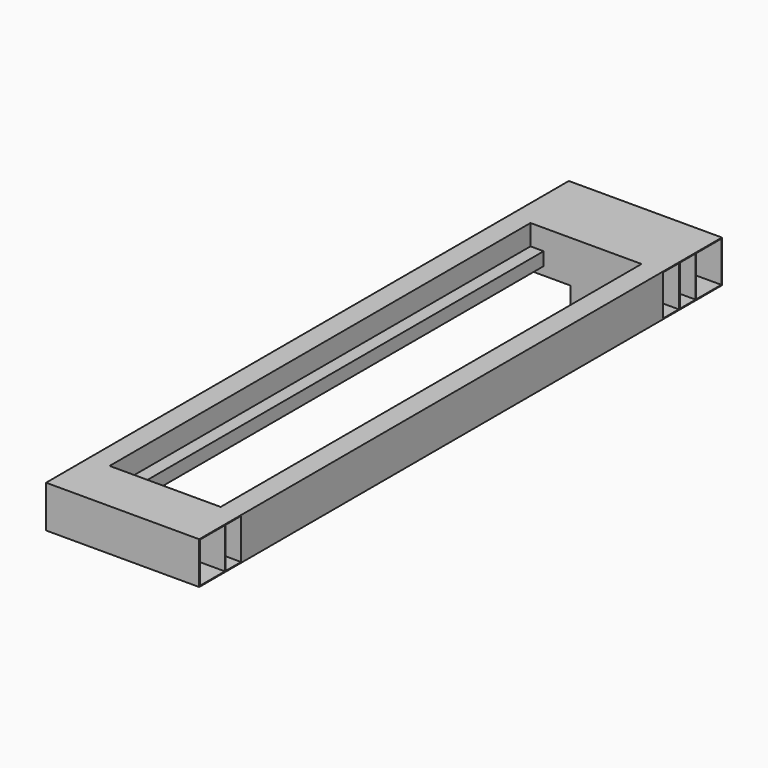
from build123d import *

# Parameters (mm, degrees)
F0_W      = 74
F0_H      = 154
F0_W_2    = 46
F0_H_2    = 46
F1_DEPTH  = 2000
F6_W      = 74
F6_H      = 154
F7_DEPTH  = 582
F8_W      = 74
F8_H      = 154
F9_DEPTH  = 582
F10_W     = 58.25
F10_H     = 30.13
F11_DEPTH = 2160.001
F12_W     = 116.5
F12_H     = 3
F13_DEPTH = 74
F14_W     = 116.5
F14_H     = 3
F15_DEPTH = 76
F16_W     = 116.5
F16_H     = 3
F17_DEPTH = 71
F18_W     = 116.5
F18_H     = 3
F19_DEPTH = 95
F20_W     = 116.5
F20_H     = 3
F20_H_2   = 22.57
F21_DEPTH = 77
F22_DEPTH = 77
F23_DEPTH = 77
F24_W     = 74
F24_H     = 154
F25_DEPTH = 582
F27_DEPTH = 3
F29_DEPTH = 582
F31_DEPTH = 25
F32_DEPTH = 582
F34_DEPTH = 25


# Not quite as in the source:
# - a feature names something its author has since deleted; it is built from what else it names


with BuildPart() as f1:
    # F0 (on Front) → F1 (new body)
    with BuildSketch(Plane.XZ):
        Polygon((-80, 0), (0, 0), (0, 16.85), (0, 31.78), (0, 81.78), (0, 160), (-77, 160), (-80, 160), align=None)
        with Locations((-40, 80)):
            Rectangle(F0_W, F0_H, mode=Mode.SUBTRACT)
        Polygon((0, 81.78), (0, 31.78), (50, 31.78), (50, 81.78), (2, 81.78), align=None)
        with Locations((25, 56.78)):
            Rectangle(F0_W_2, F0_H_2, mode=Mode.SUBTRACT)
    extrude(amount=F1_DEPTH)


with BuildPart() as f2_1:
    # F2: instance of F1
    add(f1.part.mirror(Plane(origin=(50, -1000, 56.78), x_dir=(0, 1, 0), z_dir=(1, 0, 0))))


with BuildPart() as f2_1_1:
    # F3: moved
    add(f2_1.part.moved(Location((63, 0, 0))))


with BuildPart() as f2_1_2:
    # F5: moved
    add(f2_1_1.part.moved(Location((259.1, 0, 0))))


with BuildPart() as f1_1:
    add(f1.part)

    add(f2_1_2.part)  # F7 merges F2_1
    # F6 (on face) → F7 (join)
    with BuildSketch(Plane.YZ.offset(502.1)):
        Polygon((-2000, 0), (-2000, 160), (-2077, 160), (-2080, 160), (-2080, 0), align=None)
        with Locations((-2040, 80)):
            Rectangle(F6_W, F6_H, mode=Mode.SUBTRACT)
    extrude(amount=-F7_DEPTH)

    # F8 (on face) → F9 (join)
    with BuildSketch(Plane.YZ.offset(502.1)):
        Polygon((80, 160), (0, 160), (0, 0), (3, 0), (80, 0), align=None)
        with Locations((40, 80)):
            Rectangle(F8_W, F8_H, mode=Mode.SUBTRACT)
    extrude(amount=-F9_DEPTH)

    # F10 (on face) → F11 (cut, through all)
    with BuildSketch(Plane.XZ.offset(2080)):
        with Locations((182.125, 15.065)):
            Rectangle(F10_W, F10_H)
        with Locations((240.375, 15.065)):
            Rectangle(F10_W, F10_H)
    extrude(amount=-F11_DEPTH, mode=Mode.SUBTRACT)

    # F12 (on face) + F10 (on face) → F13 (join)
    with BuildSketch(Plane(origin=(0, -2077, 0), x_dir=(-1, 0, 0), z_dir=(0, 1, 0))):
        with Locations((-211.25, 31.63)):
            Rectangle(F12_W, F12_H)
    with BuildSketch(Plane.XZ.offset(2080)):
        with Locations((182.125, 15.065)):
            Rectangle(F10_W, F10_H)
    extrude(amount=F13_DEPTH, dir=(0, 1, 0))

    # F14 (on face) → F15 (join)
    with BuildSketch(Plane.XZ.offset(-77)):
        with Locations((211.25, 31.63)):
            Rectangle(F14_W, F14_H)
    extrude(amount=F15_DEPTH)

    # F16 (on face) → F17 (join)
    with BuildSketch(Plane(origin=(0, 0, 30.13), x_dir=(1, 0, 0), z_dir=(0, 0, -1))):
        with Locations((211.25, 2001.5)):
            Rectangle(F16_W, F16_H)
    extrude(amount=F17_DEPTH)

    # F18 (on face) → F19 (join)
    with BuildSketch(Plane(origin=(0, 0, 30.13), x_dir=(1, 0, 0), z_dir=(0, 0, -1))):
        with Locations((211.25, -1.5)):
            Rectangle(F18_W, F18_H)
    extrude(amount=F19_DEPTH)

    # F20 (on face) → F21 (cut)
    with BuildSketch(Plane(origin=(0, 80, 0), x_dir=(-1, 0, 0), z_dir=(0, 1, 0))):
        with Locations((-211.25, 54.2)):
            Rectangle(F20_W, F20_H)
        with Locations((-211.25, 41.415)):
            Rectangle(F20_W, F20_H_2)
    extrude(amount=-F21_DEPTH, mode=Mode.SUBTRACT)

    # F20 (on face) → F22 (join)
    with BuildSketch(Plane(origin=(0, 80, 0), x_dir=(-1, 0, 0), z_dir=(0, 1, 0))):
        with Locations((-211.25, 54.2)):
            Rectangle(F20_W, F20_H)
    extrude(amount=-F22_DEPTH)

    # F10 (on face) → F23 (cut)
    with BuildSketch(Plane.XZ.offset(2080)):
        with Locations((182.125, 15.065)):
            Rectangle(F10_W, F10_H)
    extrude(amount=-F23_DEPTH, mode=Mode.SUBTRACT)

    # F24 (on face) → F25 (join)
    with BuildSketch(Plane(origin=(-79.9, 0, 0), x_dir=(0, -1, 0), z_dir=(-1, 0, 0))):
        Polygon((-80, 3), (-80, 160), (-160, 160), (-160, 0), (-80, 0), align=None)
        with Locations((-120, 80)):
            Rectangle(F24_W, F24_H, mode=Mode.SUBTRACT)
    extrude(amount=-F25_DEPTH)

    # F26 (on face) → F27 (join)
    with BuildSketch(Plane(origin=(0, 160, 0), x_dir=(-1, 0, 0), z_dir=(0, 1, 0))):
        Polygon((-268.7456309795, 160), (-268.7456309795, 0), (-268.7456309795, -64.9877786636), (-152.2456309795, -64.9877786636), (-152.2456309795, 160), align=None)
    extrude(amount=F27_DEPTH)

    # F28 (on face) → F29 (join)
    with BuildSketch(Plane.YZ.offset(502.1)):
        Polygon((282, 160), (160, 160), (160, 157), (279, 157), (279, 3), (160, 3), (160, 0), (282, 0), align=None)
    extrude(amount=-F29_DEPTH)

    # F30 (on face) → F31 (cut)
    with BuildSketch(Plane(origin=(0, 0, 0), x_dir=(1, 0, 0), z_dir=(0, 0, -1))):
        with BuildLine():
            ThreePointArc((250.4956309795, -222.5), (238.779902227, -194.2157287525), (210.4956309795, -182.5))
            Line((210.4956309795, -182.5), (210.4956309795, -222.5))
            Line((210.4956309795, -222.5), (210.4956309795, -262.5))
            ThreePointArc((210.4956309795, -262.5), (238.779902227, -250.7842712475), (250.4956309795, -222.5))
        make_face()
        with BuildLine():
            Line((210.4956309795, -222.5), (210.4956309795, -182.5))
            ThreePointArc((210.4956309795, -182.5), (170.4956309795, -222.5), (210.4956309795, -262.5))
            Line((210.4956309795, -262.5), (210.4956309795, -222.5))
        make_face()
    extrude(amount=-F31_DEPTH, mode=Mode.SUBTRACT)

    # F28 (on face) → F32 (join)
    with BuildSketch(Plane.YZ.offset(502.1)):
        Polygon((-2080, 157), (-2080, 160), (-2202, 160), (-2202, 0), (-2080, 0), (-2080, 3), (-2199, 3), (-2199, 157), align=None)
    extrude(amount=-F32_DEPTH)

    # F33 (on face) → F34 (cut)
    with BuildSketch(Plane(origin=(0, 0, 0), x_dir=(1, 0, 0), z_dir=(0, 0, -1))):
        with BuildLine():
            ThreePointArc((211.25, 2181), (171.25, 2141), (211.25, 2101))
            Line((211.25, 2101), (211.25, 2181))
        make_face()
        with BuildLine():
            Line((211.25, 2181), (211.25, 2101))
            ThreePointArc((211.25, 2101), (239.5342712475, 2112.7157287525), (251.25, 2141))
            ThreePointArc((251.25, 2141), (239.5342712475, 2169.2842712475), (211.25, 2181))
        make_face()
    extrude(amount=-F34_DEPTH, mode=Mode.SUBTRACT)


solid = f1_1.part
